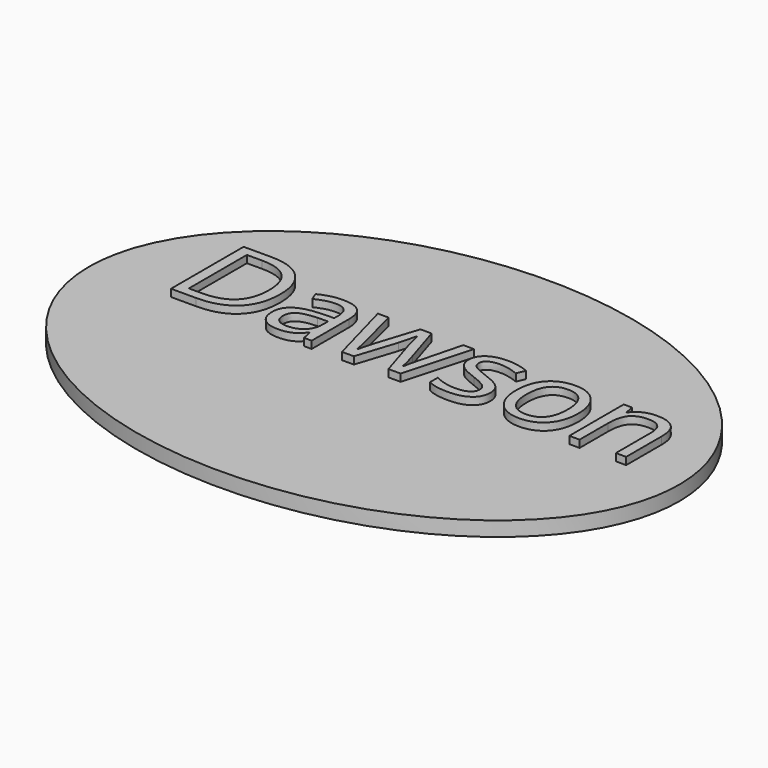
from build123d import *

# Parameters (mm, degrees)
F1_DEPTH     = 2.54
F2_TEXT_SIZE = 22.0673753776
F3_DEPTH     = 3.81


# Not quite as in the source:
# - Text() gives the source's letters only with a copy of the font that has no kerning and outlines rounded to 1/6400 em; it was checked with that copy


with BuildPart() as f1:
    # F0 (on Top) → F1 (new body)
    with BuildSketch(Plane.XY):
        with BuildLine():
            add(Edge.make_bspline(
                [(-51.2120760977, 0), (-51.2120760977, -61.9252816176), (25.6060380489, -30.9626408088), (102.4241521955, 0), (25.6060380489, 30.9626408088), (-51.2120760977, 61.9252816176), (-51.2120760977, 0)],
                knots=[0, 0, 0, 2.0943951024, 2.0943951024, 4.1887902048, 4.1887902048, 6.2831853072, 6.2831853072, 6.2831853072], degree=2, weights=[1, 0.5, 1, 0.5, 1, 0.5, 1]))
        make_face()
    extrude(amount=F1_DEPTH)

    # F2 (on Top) → F3 (join)
    with BuildSketch(Plane.XY):
        with Locations((-39.1347491572, 0)):
            Text('Dawson', F2_TEXT_SIZE, font='Open Sans', text_align=(TextAlign.LEFT, TextAlign.BOTTOM))
    extrude(amount=F3_DEPTH)


solid = f1.part
